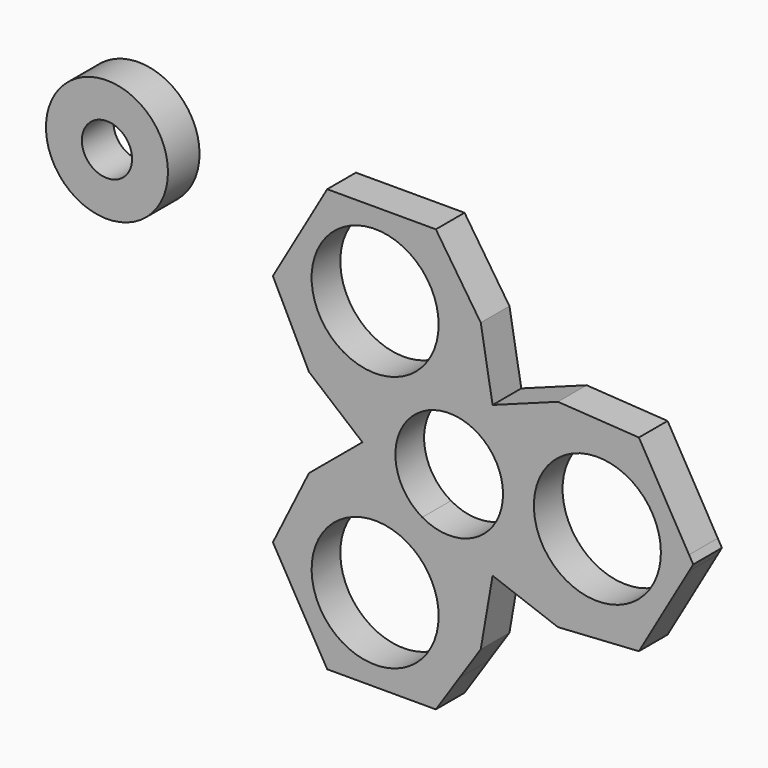
from build123d import *

# Parameters (mm, degrees)
F0_R     = 11.2395
F1_DEPTH = 6.35
F2_R     = 10.795
F2_R_2   = 4.445
F3_DEPTH = 6.985


# Not quite as in the source:
# - ends of sketch curves that miss each other by under 0.0002 mm in the source are joined


with BuildPart() as f1:
    # F0 (on Front) → F1 (new body)
    with BuildSketch(Plane.XZ):
        with BuildLine():
            Line((42.4467651581, 1.27), (33.5675281941, 16.6492895541))
            Line((33.5675281941, 16.6492895541), (19.2425445444, 17.5521669359))
            Line((19.2425445444, 17.5521669359), (7.6766035347, 13.2964561731))
            Line((7.6766035347, 13.2964561731), (5.579663063, 25.4405181745))
            Line((5.579663063, 25.4405181745), (-2.3645964913, 37.3949769354))
            Line((-2.3645964913, 37.3949769354), (-20.1235303163, 37.3949769354))
            ThreePointArc((-20.1235303163, 37.3949769354), (-21.3935303163, 37.054681461), (-22.3232348419, 36.1249769354))
            Line((-22.3232348419, 36.1249769354), (-31.2024718059, 20.7456873813))
            Line((-31.2024718059, 20.7456873813), (-31.1641125036, 20.668391129))
            Line((-31.1641125036, 20.668391129), (-27.8130050023, 13.9157122299))
            Line((-27.8130050023, 13.9157122299), (-24.8577417731, 7.960682843))
            Line((-24.8577417731, 7.960682843), (-24.8218947301, 7.8884489409))
            Line((-24.8218947301, 7.8884489409), (-15.353319828, -3.34766e-05))
            Line((-15.353319828, -3.34766e-05), (-24.8219665561, -7.8881291301))
            Line((-24.8219665561, -7.8881291301), (-24.8578663434, -7.9604670809))
            Line((-24.8578663434, -7.9604670809), (-31.1643564099, -20.6680233587))
            Line((-31.1643564099, -20.6680233587), (-31.2027017544, -20.7452890988))
            Line((-31.2027017544, -20.7452890988), (-22.3232348418, -36.1249769356))
            ThreePointArc((-22.3232348418, -36.1249769356), (-21.9195815404, -36.6510281597), (-21.3935303163, -37.0546814611))
            ThreePointArc((-21.3935303163, -37.0546814611), (-20.7809306909, -37.3084285342), (-20.1235303165, -37.3949769354))
            Line((-20.1235303165, -37.3949769354), (-2.3645964913, -37.3949769354))
            Line((-2.3645964913, -37.3949769354), (-2.3168550697, -37.3231360229))
            Line((-2.3168550697, -37.3231360229), (1.8552556307, -31.0449769354))
            Line((1.8552556307, -31.0449769354), (5.579663063, -25.4405181745))
            Line((5.579663063, -25.4405181745), (7.6765207659, -13.2964418818))
            Line((7.6765207659, -13.2964418818), (19.2425445444, -17.5521669359))
            Line((19.2425445444, -17.5521669359), (25.957862804, -17.1289127727))
            Line((25.957862804, -17.1289127727), (33.5675281941, -16.6492895541))
            Line((33.5675281941, -16.6492895541), (42.4467651581, -1.27))
            ThreePointArc((42.4467651581, -1.27), (42.7870606325, 0), (42.4467651581, 1.27))
        make_face()
        with BuildLine():
            ThreePointArc((-1.8702560234, -22.7067635073), (-22.8434485492, -28.3265135073), (-7.4900060234, -12.9730709815))
            ThreePointArc((-7.4900060234, -12.9730709815), (-3.3760634975, -17.0870135073), (-1.8702560234, -22.7067635073))
        make_face(mode=Mode.SUBTRACT)
        with BuildLine():
            ThreePointArc((-4.7625, -8.248891971), (-4.7625, 8.248891971), (9.525, 0))
            ThreePointArc((9.525, 0), (4.7625, -8.248891971), (-4.7625, -8.248891971))
        make_face(mode=Mode.SUBTRACT)
        with Locations((-13.1097560234, 22.7067635073)):
            Circle(F0_R, mode=Mode.SUBTRACT)
        with Locations((26.2195120463, 0.0001612286)):
            Circle(F0_R, mode=Mode.SUBTRACT)
        with BuildLine():
            Line((43.18, 0), (42.4467651581, 1.27))
            ThreePointArc((42.4467651581, 1.27), (42.7870606325, 0), (42.4467651581, -1.27))
            Line((42.4467651581, -1.27), (43.18, 0))
        make_face()
        with BuildLine():
            ThreePointArc((-22.3232348419, 36.1249769354), (-21.3935303163, 37.054681461), (-20.1235303163, 37.3949769354))
            Line((-20.1235303163, 37.3949769354), (-21.59, 37.3949769354))
            Line((-21.59, 37.3949769354), (-22.3232348419, 36.1249769354))
        make_face()
        with BuildLine():
            Line((-21.59, -37.3949769354), (-20.1235303165, -37.3949769354))
            ThreePointArc((-20.1235303165, -37.3949769354), (-20.7809306909, -37.3084285342), (-21.3935303163, -37.0546814611))
            Line((-21.3935303163, -37.0546814611), (-21.59, -37.3949769354))
        make_face()
        with BuildLine():
            Line((-21.59, -37.3949769354), (-21.3935303163, -37.0546814611))
            ThreePointArc((-21.3935303163, -37.0546814611), (-21.9195815404, -36.6510281597), (-22.3232348418, -36.1249769356))
            Line((-22.3232348418, -36.1249769356), (-21.59, -37.3949769354))
        make_face()
    extrude(amount=F1_DEPTH)


with BuildPart() as f3:
    # F2 (on Front) → F3 (new body)
    with BuildSketch(Plane.XZ):
        with Locations((-60.0547902286, 31.3041508198)):
            Circle(F2_R)
        with Locations((-60.0547902286, 31.3041508198)):
            Circle(F2_R_2, mode=Mode.SUBTRACT)
    extrude(amount=F3_DEPTH)


solid = Compound([f1.part, f3.part])
